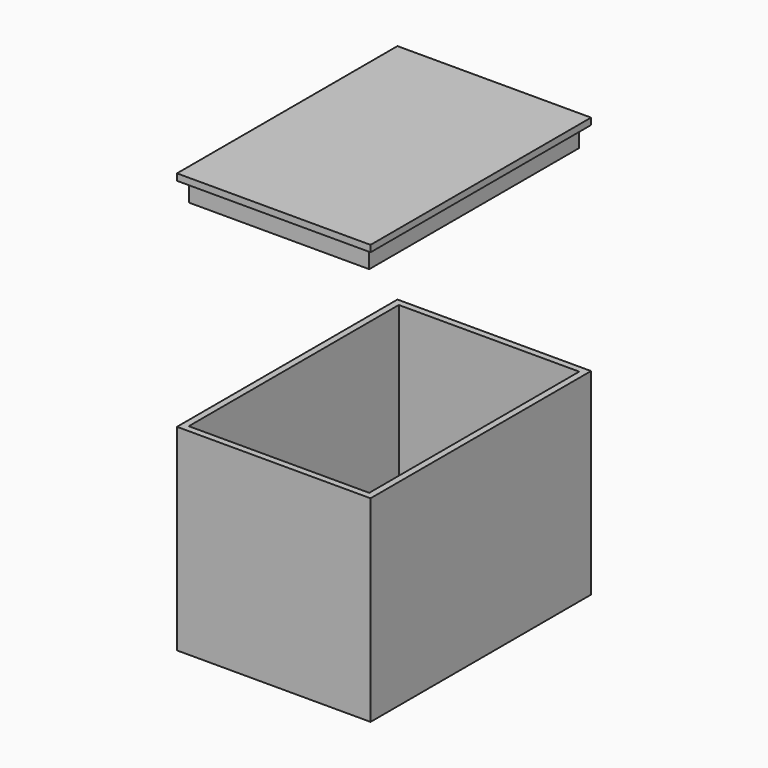
from build123d import *

# Parameters (mm, degrees)
F0_W      = 55
F0_H      = 80
F1_DEPTH  = 2
F0_W_2    = 58.9999967363
F0_H_2    = 83.9999967363
F2_DEPTH  = 60
F3_START  = 120
F1_FACE_W = 55
F1_FACE_H = 80
F3_DEPTH  = 6
F4_START  = 126
F4_DEPTH  = 2
F5_R      = 3.395090495
F5_W      = 40.5
F5_H      = 34.5
F6_DEPTH  = 16.7


# Not quite as in the source:
# - a feature names something its author has since deleted; it is built from what else it names


with BuildPart() as f1:
    # F0 (on Top) → F1 (new body)
    with BuildSketch(Plane.XY):
        with Locations((-0.6564213149, 6.3218075262)):
            Rectangle(F0_W, F0_H)
    extrude(amount=F1_DEPTH)

    # F0 (on Top) → F2 (join)
    with BuildSketch(Plane.XY):
        with Locations((-0.6564213149, 6.3218075262)):
            Rectangle(F0_W_2, F0_H_2)
        with Locations((-0.6564213149, 6.3218075262)):
            Rectangle(F0_W, F0_H, mode=Mode.SUBTRACT)
    extrude(amount=F2_DEPTH)

    # F5 (on face) → F6 (cut)
    with BuildSketch(Plane.XY):
        with Locations((-0.6564213149, -15.506147407)):
            Circle(F5_R)
        with Locations((-0.6564213149, 15.7543346533)):
            Rectangle(F5_W, F5_H)
    extrude(amount=F6_DEPTH, mode=Mode.SUBTRACT)


with BuildPart() as f3:
    # F1_face (on face) + F0 (on Top) → F3 (new body)
    with BuildSketch(Plane(origin=(-0.6564213149, 6.3218075262, 2), x_dir=(1, 0, 0), z_dir=(0, 0, 1)).offset(F3_START)):
        Rectangle(F1_FACE_W, F1_FACE_H)
    with BuildSketch(Plane.XY.offset(F3_START)):
        with Locations((-0.6564213149, 6.3218075262)):
            Rectangle(F0_W, F0_H)
    extrude(amount=F3_DEPTH)

    # F0 (on Top) → F4 (join)
    with BuildSketch(Plane.XY.offset(F4_START)):
        with Locations((-0.6564213149, 6.3218075262)):
            Rectangle(F0_W_2, F0_H_2)
        with Locations((-0.6564213149, 6.3218075262)):
            Rectangle(F0_W, F0_H, mode=Mode.SUBTRACT)
    extrude(amount=F4_DEPTH)


solid = Compound([f1.part, f3.part])
